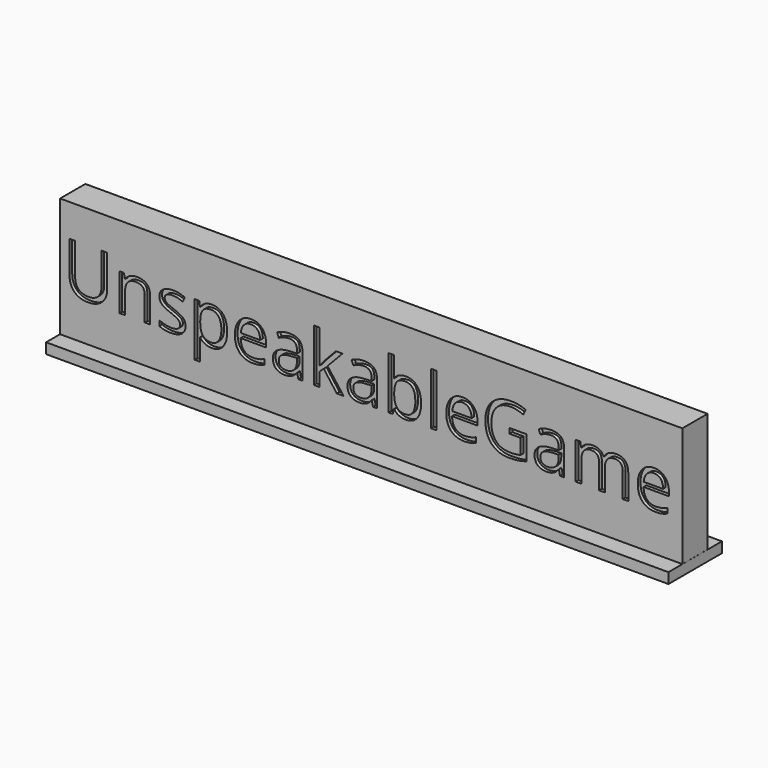
from build123d import *

# Parameters (mm, degrees)
F0_W         = 185.42
F0_H         = 35.6108
F1_DEPTH     = 9.398
F2_TEXT_SIZE = 20.5613963772
F3_DEPTH     = 1.016
F4_W         = 185.4563206434
F4_H         = 19.9183849618
F4_W_2       = 185.42
F4_H_2       = 9.398
F5_DEPTH     = 3.1242


# Not quite as in the source:
# - Text() gives the source's letters only with a copy of the font that has no kerning and outlines rounded to 1/6400 em; it was checked with that copy


with BuildPart() as f1:
    # F0 (on Front) → F1 (new body)
    with BuildSketch(Plane.XZ):
        Rectangle(F0_W, F0_H)
    extrude(amount=F1_DEPTH)

    # F2 (on face) → F3 (cut)
    with BuildSketch(Plane.XZ.offset(9.398)):
        with Locations((-91.7860860936, -6.5273091313)):
            Text('UnspeakableGame', F2_TEXT_SIZE, font='Open Sans', text_align=(TextAlign.LEFT, TextAlign.BOTTOM))
    extrude(amount=-F3_DEPTH, mode=Mode.SUBTRACT)

    # F4 (on face) → F5 (join)
    with BuildSketch(Plane(origin=(0, 0, -17.8054), x_dir=(1, 0, 0), z_dir=(0, 0, -1))):
        with Locations((0, 4.6431371011)):
            Rectangle(F4_W, F4_H)
        with Locations((0, 4.699)):
            Rectangle(F4_W_2, F4_H_2, mode=Mode.SUBTRACT)
        with Locations((0, 4.699)):
            Rectangle(F4_W_2, F4_H_2)
    extrude(amount=F5_DEPTH)


solid = f1.part
